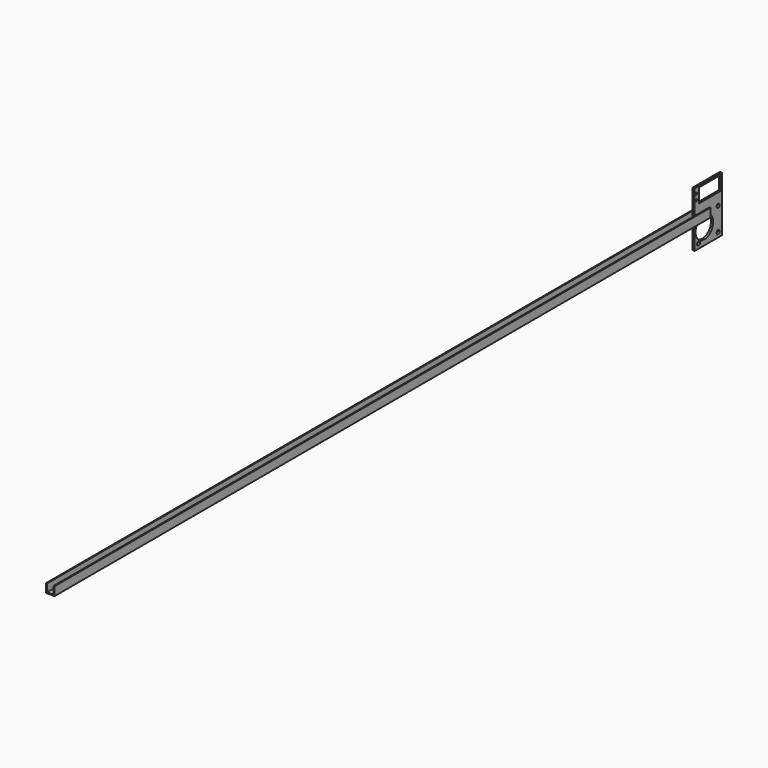
from build123d import *

# Parameters (mm, degrees)
F1_DEPTH = 1219.2
F2_W     = 50.5127292126
F2_H     = 82.0375010371
F2_R     = 2.89913405
F2_R_2   = 2.8318920873
F2_R_3   = 2.8588761336
F2_R_4   = 1.5183628154
F2_R_5   = 1.4519166982
F2_R_6   = 2.8173846153
F2_W_2   = 41.0130396485
F2_H_2   = 20.9737662226
F3_DEPTH = 3.06
F5_R     = 16.3147290841
F6_DEPTH = 5


with BuildPart() as f1:
    # F0 (on Front) → F1 (new body)
    with BuildSketch(Plane.XZ):
        Polygon((-4.825, 6.5), (-6.325, 6.5), (-6.325, -6.5), (6.325, -6.5), (6.325, 6.5), (4.825, 6.5), (4.825, -5), (-4.825, -5), align=None)
    extrude(amount=F1_DEPTH)


with BuildPart() as f3:
    # F2 (on Right) → F3 (new body)
    with BuildSketch(Plane.YZ):
        with Locations((0.0250553712, 0.0057928264)):
            Rectangle(F2_W, F2_H)
        with Locations((-18.1433722998, -33.8706020266)):
            Circle(F2_R, mode=Mode.SUBTRACT)
        with Locations((18.2029870339, -33.8714673854)):
            Circle(F2_R_2, mode=Mode.SUBTRACT)
        with Locations((-18.0760649964, 0.4261299481)):
            Circle(F2_R_3, mode=Mode.SUBTRACT)
        with Locations((-22.3539447378, 23.9319726942)):
            Circle(F2_R_4, mode=Mode.SUBTRACT)
        with Locations((-22.3546241195, 32.8359914765)):
            Circle(F2_R_5, mode=Mode.SUBTRACT)
        with Locations((18.1693327613, 0.3677118686)):
            Circle(F2_R_6, mode=Mode.SUBTRACT)
        with Locations((2.7500502765, 28.4059746191)):
            Rectangle(F2_W_2, F2_H_2, mode=Mode.SUBTRACT)
    extrude(amount=F3_DEPTH)

    # F5 (on face) → F6 (cut)
    with BuildSketch(Plane.YZ.offset(3.06)):
        with Locations((-7.363283649, -16.781862238)):
            Circle(F5_R)
    extrude(amount=-F6_DEPTH, mode=Mode.SUBTRACT)


solid = Compound([f1.part, f3.part])
